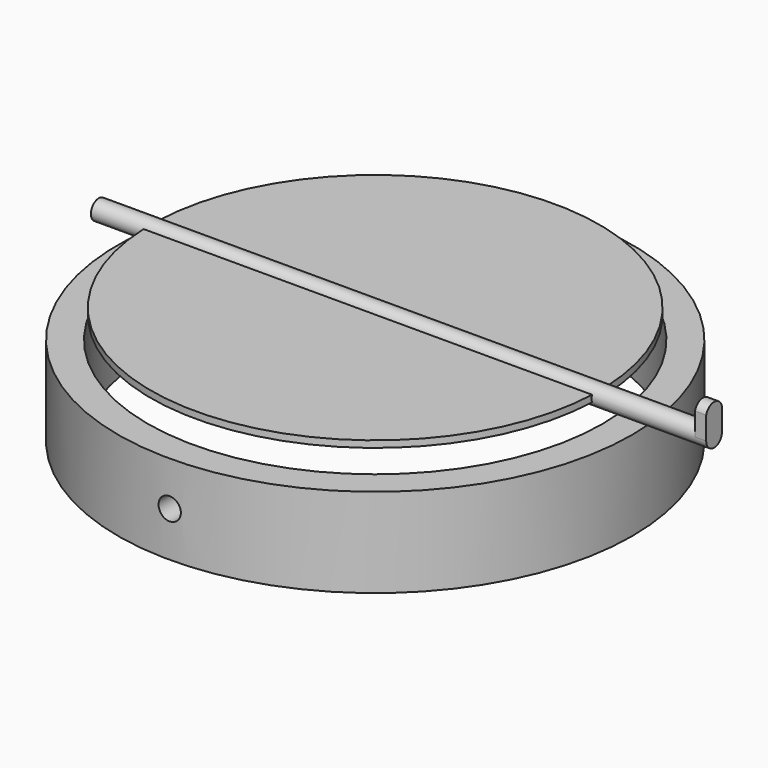
from build123d import *

# Parameters (mm, degrees)
F2_R      = 45.8267789271
F0_R      = 28.6708469649
F4_T      = -2.5
F9_R      = 28.8324086219
F9_R_2    = 25.5072919531
F10_DEPTH = 5
F11_R     = 1.25
F12_DEPTH = 28.8334086219
F13_DEPTH = 31
F14_R     = 25.1680354712
F15_DEPTH = 0.375
F16_R     = 1.1
F17_DEPTH = 38
F18_DEPTH = 31
F20_DEPTH = 1.25


# Not quite as in the source:
# - a feature of the source that left no trace in its solid (it failed there, or was rolled back) is left out


with BuildPart() as f3:
    # F2 (on offset) → F3 section 0
    with BuildSketch(Plane.XY.offset(140)):
        with Locations((0, 0.2770116553)):
            Circle(F2_R)
    # F0 (on Top) → F3 section 1
    with BuildSketch(Plane.XY):
        with Locations((0, -0.2653934062)):
            Circle(F0_R)
    loft()

    # F4
    f4_openings = [f3.faces().sort_by_distance(p)[0] for p in [
        (0, 0.277012, 140),
        (0, -0.265393, 0),
    ]]
    offset(amount=F4_T, openings=f4_openings)


with BuildPart() as f10:
    # F9 (on offset) → F10 (new body, symmetric)
    with BuildSketch(Plane.XY.offset(-7.8)):
        Circle(F9_R)
        Circle(F9_R_2, mode=Mode.SUBTRACT)
    extrude(amount=F10_DEPTH, both=True)

    # F11 (on Front) → F12 (cut, through all)
    with BuildSketch(Plane.XZ):
        with Locations((0, -7.7568855078)):
            Circle(F11_R)
    extrude(amount=F12_DEPTH, mode=Mode.SUBTRACT)

    # F11 (on Front) → F13 (cut)
    with BuildSketch(Plane.XZ):
        with Locations((0, -7.7568855078)):
            Circle(F11_R)
    extrude(amount=-F13_DEPTH, mode=Mode.SUBTRACT)


with BuildPart() as f15:
    # F14 (on Top) → F15 (new body, symmetric)
    with BuildSketch(Plane.XY):
        Circle(F14_R)
    extrude(amount=F15_DEPTH, both=True)

    # F16 (on Right) → F17 (join)
    with BuildSketch(Plane.YZ):
        Circle(F16_R)
    extrude(amount=F17_DEPTH)

    # F16 (on Right) → F18 (join)
    with BuildSketch(Plane.YZ):
        Circle(F16_R)
    extrude(amount=-F18_DEPTH)

    # F19 (on face) → F20 (join)
    with BuildSketch(Plane.YZ.offset(38)):
        with BuildLine():
            Line((-1.1, 2.5760282297), (-1.1, 0))
            ThreePointArc((-1.1, 0), (0, 1.1), (1.1, 0))
            Line((1.1, 0), (1.1020586826, 0))
            Line((1.1020586826, 0), (1.1020586826, 2.5760282297))
            ThreePointArc((1.1020586826, 2.5760282297), (0.0010293413, 3.4287400368), (-1.1, 2.5760282297))
        make_face()
        with BuildLine():
            ThreePointArc((1.1, 0), (0, 1.1), (-1.1, 0))
            Line((-1.1, 0), (1.1, 0))
        make_face()
    extrude(amount=-F20_DEPTH)


solid = Compound([f10.part, f15.part])
